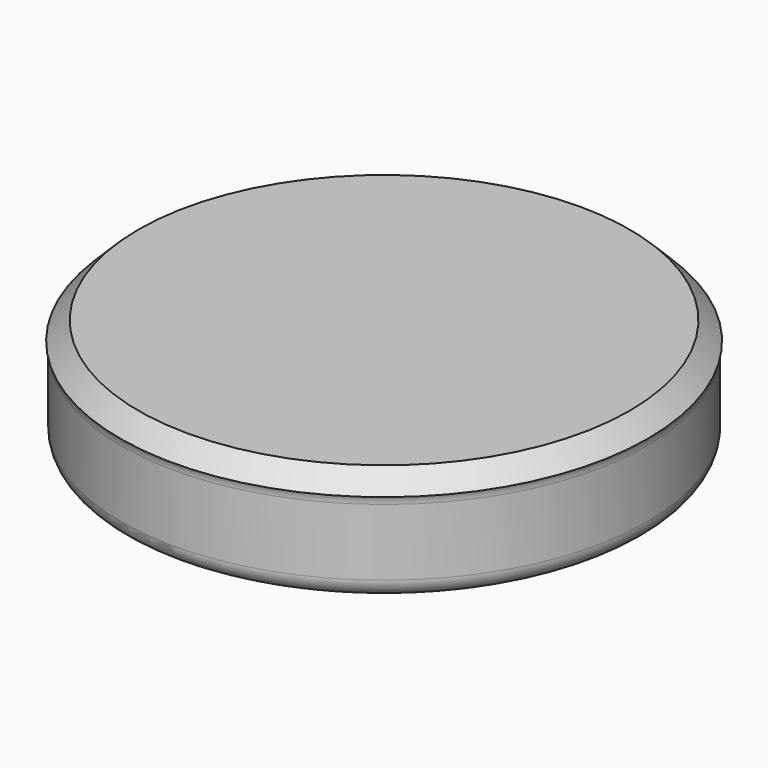
from build123d import *

# Parameters (mm, degrees)
F2_R     = 71.4411374157
F3_DEPTH = 5
F4_R     = 71.0302069346
F6_DEPTH = 25
F7_R     = 0.0241421356


# Not quite as in the source:
# - a fillet or chamfer that OpenCascade refuses, or shapes differently, is made with other operations: its cross-section is extruded or revolved along the edge and cut away or added


with BuildPart() as f3:
    # F2 (on Top) → F3 (new body)
    with BuildSketch(Plane.XY):
        Circle(F2_R)
    extrude(amount=F3_DEPTH)

    # F4 (on face) → F6 (join)
    with BuildSketch(Plane(origin=(0, 0, 0), x_dir=(1, 0, 0), z_dir=(0, 0, -1))):
        Circle(F4_R)
    extrude(amount=F6_DEPTH)

    # F7
    f7_edges = [f3.edges().sort_by_distance(p)[0] for p in [
        (-71.441137, 0, 0),
    ]]
    fillet(f7_edges, radius=F7_R)

    # F8: chamfer of 5 on 1 edges, made by hand

    # F8_s1 → F8_t2 (revolve, cut)
    with BuildSketch(Plane.XZ):
        Polygon((71.4411374157, 0), (66.4411374157, 5), (71.4411374157, 5), align=None)
    revolve(axis=Axis((0, 0, 5), (0, 0, 1)), mode=Mode.SUBTRACT)

    # F9: fillet of radius 5 on 3 edges, made by hand

    # F9_s1 → F9_t2 (revolve, cut)
    with BuildSketch(Plane.XZ):
        with BuildLine():
            ThreePointArc((71.0302069346, -20), (69.5657408405, -23.5355339059), (66.0302069346, -25))
            Line((66.0302069346, -25), (66.0302069346, -25.1))
            Line((66.0302069346, -25.1), (71.1302069346, -25.1))
            Line((71.1302069346, -25.1), (71.1302069346, -20))
            Line((71.1302069346, -20), (71.0302069346, -20))
        make_face()
    revolve(axis=Axis((0, 0, -25), (0, 0, -1)), mode=Mode.SUBTRACT)

    # F9_s3 → F9_t4 (revolve)
    with BuildSketch(Plane.XZ):
        with BuildLine():
            ThreePointArc((71.4340663479, 0.0070710678), (71.1322122973, -0.9567431048), (71.0302069346, -1.9615557905))
            Line((71.0302069346, -1.9615557905), (70.9302069346, -1.9615557905))
            Line((70.9302069346, -1.9615557905), (70.9302069346, 0))
            Line((70.9302069346, 0), (71.0302069346, 0.1))
            ThreePointArc((71.0302069346, 0.1), (71.2321366412, 0.1), (71.3421435362, 0.046443605))
            Line((71.3421435362, 0.046443605), (71.4340663479, 0.0070710678))
        make_face()
    revolve(axis=Axis((0, 0, 0), (0, 0, -1)))


solid = f3.part
